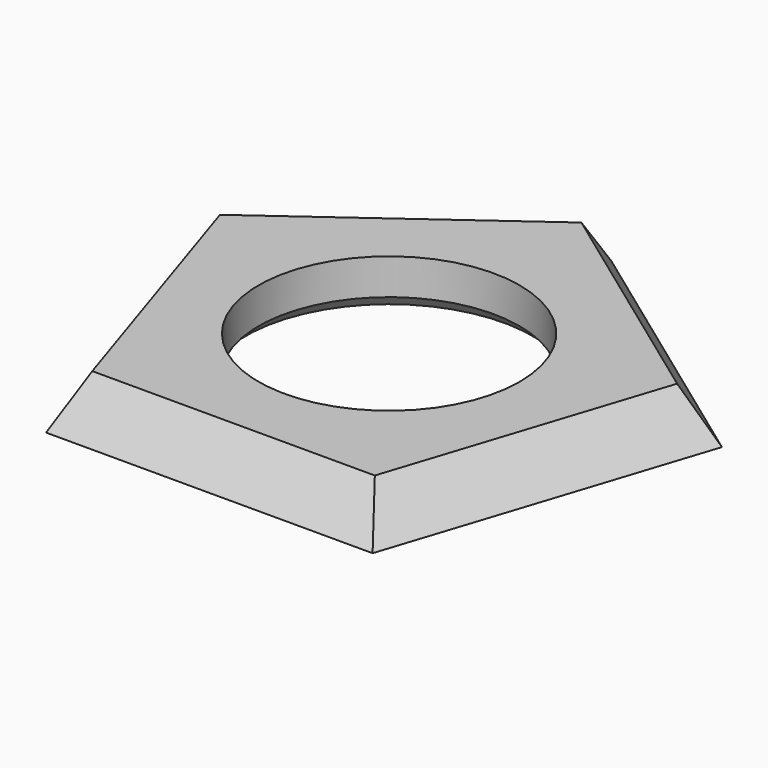
from build123d import *

# Parameters (mm, degrees)
F0_R     = 50.8
F1_DEPTH = 19.05
F2_SIZE2 = 11.76551
F2_SIZE  = 19.04999
F3_SIZE  = 5.08


# Not quite as in the source:
# - a fillet or chamfer is up to 0.001 mm smaller than in the source, because OpenCascade refuses the exact size


with BuildPart() as f1:
    # F0 (on Top) → F1 (new body)
    with BuildSketch(Plane.XY):
        Polygon((0, 108.0326526607), (-102.7451582856, 33.3839256196), (-63.5, -87.4002519499), (63.5, -87.4002519499), (102.7451582856, 33.3839256196), align=None)
        Circle(F0_R, mode=Mode.SUBTRACT)
    extrude(amount=F1_DEPTH)

    # F2 (size 19.05 and 11.7655197988 in the source; OpenCascade refuses exactly that, so slightly less here)
    f2_edges = [f1.edges().sort_by_distance(p)[0] for p in [
        (0, -87.400252, 19.05),
        (83.122579, -27.008163, 19.05),
        (51.372579, 70.708289, 19.05),
        (-51.372579, 70.708289, 19.05),
        (-83.122579, -27.008163, 19.05),
    ]]
    chamfer(f2_edges, length=F2_SIZE, length2=F2_SIZE2)

    # F3
    f3_edges = [f1.edges().sort_by_distance(p)[0] for p in [
        (-50.8, 0, 0),
    ]]
    chamfer(f3_edges, length=F3_SIZE)


solid = f1.part
